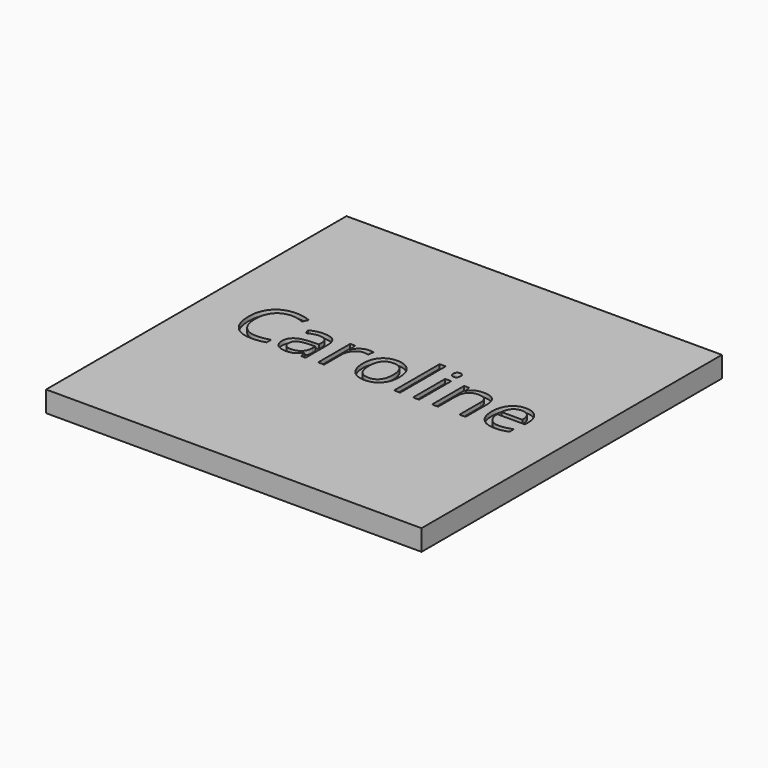
from build123d import *

# Parameters (mm, degrees)
F0_W         = 90
F0_H         = 90
F1_DEPTH     = 5
F2_TEXT_SIZE = 17.9825793762
F3_DEPTH     = 1


# Not quite as in the source:
# - Text() gives the source's letters only with a copy of the font that has no kerning and outlines rounded to 1/6400 em; it was checked with that copy


with BuildPart() as f1:
    # F0 (on Top) → F1 (new body)
    with BuildSketch(Plane.XY):
        Rectangle(F0_W, F0_H)
    extrude(amount=F1_DEPTH)

    # F2 (on face) → F3 (cut)
    with BuildSketch(Plane.XY.offset(5)):
        with Locations((-35, -4.6114230185)):
            Text('Caroline', F2_TEXT_SIZE, font='Open Sans', text_align=(TextAlign.LEFT, TextAlign.BOTTOM))
    extrude(amount=-F3_DEPTH, mode=Mode.SUBTRACT)


solid = f1.part
